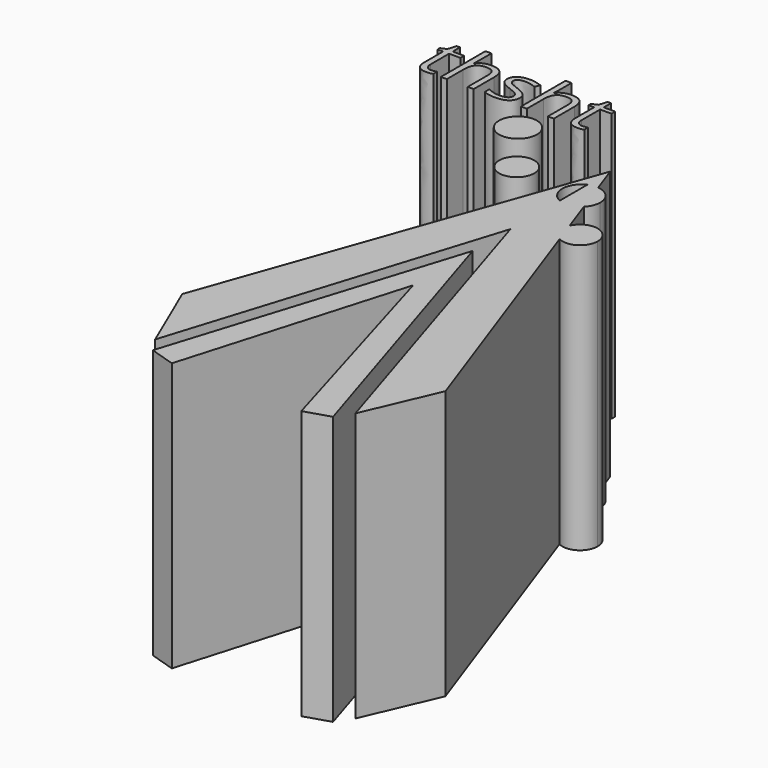
from build123d import *

# Parameters (mm, degrees)
F0_R         = 1.633150864
F0_R_2       = 1.7617151423
F0_TEXT_SIZE = 6.8324734457
F1_DEPTH     = 25


# Not quite as in the source:
# - Text() gives the source's letters only with a copy of the font that has no kerning and outlines rounded to 1/6400 em; it was checked with that copy


with BuildPart() as f1:
    # F0 (on Top) → F1 (new body)
    with BuildSketch(Plane.XY):
        Polygon((-3.2559314023, -37.9656802242), (-11.6436841143, -11.2365347827), (-11.6436841143, -18.1588975263), (-5.6186615524, -38.7071179281), align=None)
        Polygon((-11.6436841143, -18.1588975263), (-11.6436841143, -11.2365347827), (-20.0314368262, -37.9656802242), (-17.6687066761, -38.7071179281), align=None)
        with BuildLine():
            Line((-20.9621969731, -36.5344271097), (-11.6436841143, -6.8392400848))
            Line((-11.6436841143, -6.8392400848), (-11.6436841143, -1.1113375246))
            ThreePointArc((-11.6436841143, -1.1113375246), (-12.6786187573, 0.4934772151), (-11.6436841143, 2.0982919547))
            Line((-11.6436841143, 2.0982919547), (-11.6436841143, 4.7630163338))
            Line((-11.6436841143, 4.7630163338), (-23.8899588585, -29.7128986567))
            Line((-23.8899588585, -29.7128986567), (-20.9621969731, -36.5344271097))
        make_face()
        with BuildLine():
            Line((-11.6436841143, -1.1113375246), (-11.6436841143, -6.8392400848))
            Line((-11.6436841143, -6.8392400848), (-2.3251712555, -36.5344271097))
            Line((-2.3251712555, -36.5344271097), (0.60259063, -29.7128986567))
            Line((0.60259063, -29.7128986567), (-7.8775300928, -5.839522691))
            ThreePointArc((-7.8775300928, -5.839522691), (-8.6638824666, -4.9367665501), (-8.6232199101, -3.7402443973))
            Line((-8.6232199101, -3.7402443973), (-9.6811001582, -0.7620824446))
            ThreePointArc((-9.6811001582, -0.7620824446), (-10.6082438176, -1.2409879394), (-11.6436841143, -1.1113375246))
        make_face()
        with BuildLine():
            Line((-11.6436841143, 2.0982919547), (-11.6436841143, -1.1113375246))
            ThreePointArc((-11.6436841143, -1.1113375246), (-10.6082438176, -1.2409879394), (-9.6811001582, -0.7620824446))
            Line((-9.6811001582, -0.7620824446), (-10.7500611467, 2.2472741912))
            ThreePointArc((-10.7500611467, 2.2472741912), (-11.2066130838, 2.2312081109), (-11.6436841143, 2.0982919547))
        make_face()
        with BuildLine():
            Line((-11.6436841143, 4.7630163338), (-11.6436841143, 2.0982919547))
            ThreePointArc((-11.6436841143, 2.0982919547), (-11.2066130838, 2.2312081109), (-10.7500611467, 2.2472741912))
            Line((-10.7500611467, 2.2472741912), (-11.6436841143, 4.7630163338))
        make_face()
        with BuildLine():
            Line((-10.7500611467, 2.2472741912), (-9.6811001582, -0.7620824446))
            ThreePointArc((-9.6811001582, -0.7620824446), (-9.291976862, -0.1871499149), (-9.1551884727, 0.4934772151))
            ThreePointArc((-9.1551884727, 0.4934772151), (-9.6135293124, 1.6787432906), (-10.7500611467, 2.2472741912))
        make_face()
        with BuildLine():
            ThreePointArc((-5.4917862755, -4.390113987), (-6.7930787787, -2.7910355734), (-8.6232199101, -3.7402443973))
            Line((-8.6232199101, -3.7402443973), (-7.8775300928, -5.839522691))
            ThreePointArc((-7.8775300928, -5.839522691), (-6.2769737226, -5.7858717699), (-5.4917862755, -4.390113987))
        make_face()
        with BuildLine():
            Line((-7.8775300928, -5.839522691), (-8.6232199101, -3.7402443973))
            ThreePointArc((-8.6232199101, -3.7402443973), (-8.6638824666, -4.9367665501), (-7.8775300928, -5.839522691))
        make_face()
        with Locations((-17.4092068337, 1.0967458948)):
            Circle(F0_R)
        with Locations((-21.2011733092, 5.9803370968)):
            Circle(F0_R_2)
        with Locations((-33.5570089519, 8.7030371651)):
            Text('thsht', F0_TEXT_SIZE, font='Open Sans', text_align=(TextAlign.LEFT, TextAlign.BOTTOM))
    extrude(amount=F1_DEPTH)


solid = f1.part
